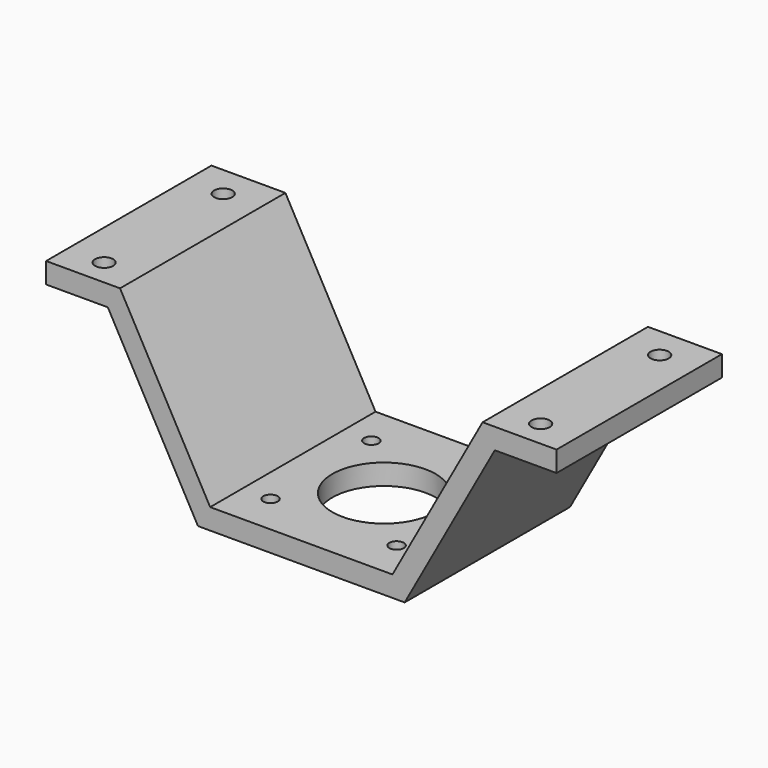
from build123d import *

# Parameters (mm, degrees)
F0_W     = 50
F0_H     = 50
F0_R     = 1.75
F0_R_2   = 12.5
F1_DEPTH = 5
F3_DEPTH = 50
F5_D     = 4.4


with BuildPart() as f1:
    # F0 (on Top) → F1 (new body)
    with BuildSketch(Plane.XY):
        Rectangle(F0_W, F0_H)
        with Locations((-15.25, -15.25)):
            Circle(F0_R, mode=Mode.SUBTRACT)
        with Locations((15.25, -15.25)):
            Circle(F0_R, mode=Mode.SUBTRACT)
        with Locations((-15.25, 15.25)):
            Circle(F0_R, mode=Mode.SUBTRACT)
        Circle(F0_R_2, mode=Mode.SUBTRACT)
        with Locations((15.25, 15.25)):
            Circle(F0_R, mode=Mode.SUBTRACT)
    extrude(amount=F1_DEPTH)

    # F2 (on face) → F3 (join, through all)
    with BuildSketch(Plane.XZ.offset(25)):
        Polygon((-46.7986041229, 39.5), (-25, 0), (-25, 5), (-22.0484650111, 5), (-43.847069134, 44.5), (-61.7379361051, 44.5), (-61.7379361051, 39.5), align=None)
        Polygon((25, 5), (25, 0), (46.7986041229, 39.5), (61.7379361051, 39.5), (61.7379361051, 44.5), (43.847069134, 44.5), (22.0484650111, 5), align=None)
    extrude(amount=-F3_DEPTH)

    # F5 (through all)
    with Locations(Plane.XY.offset(44.5)):
        with Locations((-52.7925026196, 17.3637714833), (-52.7925026196, -18.6362285167), (52.7925026196, -18.6362285167), (52.7925026196, 17.3637714833)):
            Hole(F5_D / 2)


solid = f1.part
